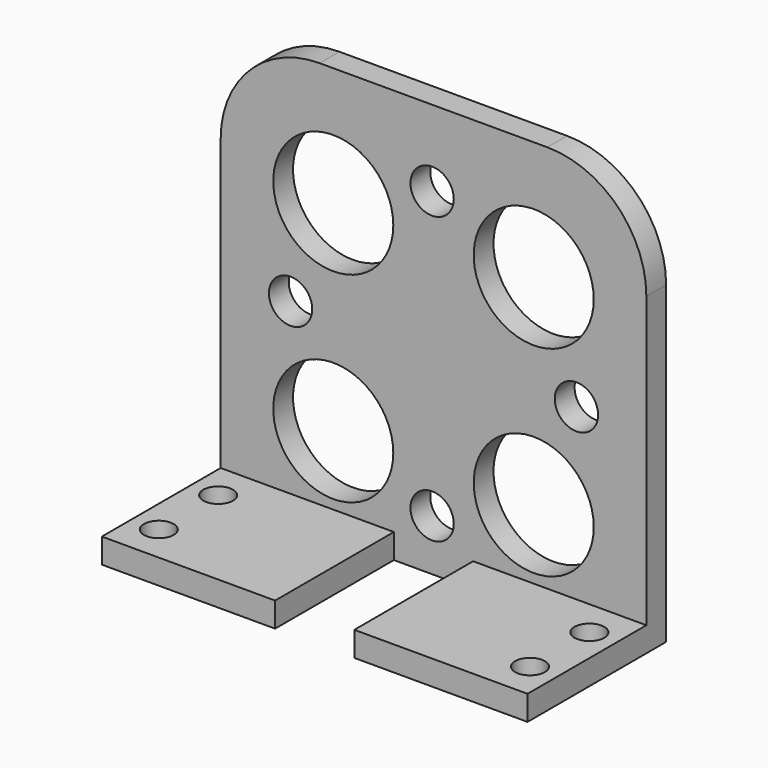
from build123d import *

# Parameters (mm, degrees)
F0_R     = 1.75
F0_R_2   = 4.85
F1_DEPTH = 2
F2_W     = 14
F2_H     = 2
F3_DEPTH = 12
F5_D     = 2.4


# Not quite as in the source:
# - a feature names something its author has since deleted; it is built from what else it names


with BuildPart() as f1:
    # F0 (on Front) → F1 (new body)
    with BuildSketch(Plane.XZ):
        with BuildLine():
            Line((9.2, 17.7), (-9.2, 17.7))
            ThreePointArc((-9.2, 17.7), (-14.8568542495, 15.3568542495), (-17.2, 9.7))
            Line((-17.2, 9.7), (-17.2, -15.7))
            Line((-17.2, -15.7), (17.2, -15.7))
            Line((17.2, -15.7), (17.2, 9.7))
            ThreePointArc((17.2, 9.7), (14.8568542495, 15.3568542495), (9.2, 17.7))
        make_face()
        with Locations((-0.1129766364, -11.55)):
            Circle(F0_R, mode=Mode.SUBTRACT)
        with Locations((-8.1, -8.1)):
            Circle(F0_R_2, mode=Mode.SUBTRACT)
        with Locations((-11.55, 0)):
            Circle(F0_R, mode=Mode.SUBTRACT)
        with Locations((8.1, -8.1)):
            Circle(F0_R_2, mode=Mode.SUBTRACT)
        with Locations((11.55, 0)):
            Circle(F0_R, mode=Mode.SUBTRACT)
        with Locations((-8.1, 8.1)):
            Circle(F0_R_2, mode=Mode.SUBTRACT)
        with Locations((-0.1129766364, 11.55)):
            Circle(F0_R, mode=Mode.SUBTRACT)
        with Locations((8.1, 8.1)):
            Circle(F0_R_2, mode=Mode.SUBTRACT)
    extrude(amount=F1_DEPTH)

    # F2 (on face) → F3 (join)
    with BuildSketch(Plane.XZ.offset(2)):
        with Locations((-10.2, -14.7)):
            Rectangle(F2_W, F2_H)
        with Locations((10.2, -14.7)):
            Rectangle(F2_W, F2_H)
    extrude(amount=F3_DEPTH)

    # F5 (through all)
    with Locations(Plane(origin=(0, 0, -15.7), x_dir=(1, 0, 0), z_dir=(0, 0, -1))):
        with Locations((-15, 11), (-15, 5), (15, 11), (15, 5)):
            Hole(F5_D / 2)


solid = f1.part
